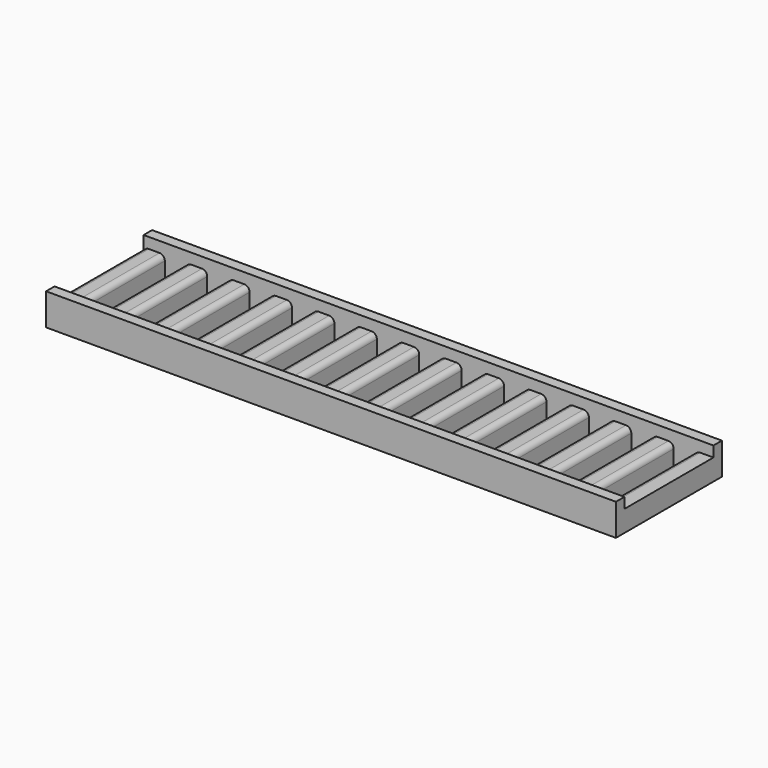
from build123d import *

# Parameters (mm, degrees)
F0_W     = 107.5
F0_H     = 25
F0_W_2   = 4
F0_H_2   = 21
F1_DEPTH = 4
F2_R     = 1
F3_W     = 107.5
F3_H     = 2
F4_DEPTH = 2
F5_R     = 1


# Not quite as in the source:
# - a feature names something its author has since deleted; it is built from what else it names


with BuildPart() as f1:
    # F0 (on Top) → F1 (new body)
    with BuildSketch(Plane.XY):
        with Locations((53.75, 12.5)):
            Rectangle(F0_W, F0_H)
        with Locations((6, 12.5)):
            Rectangle(F0_W_2, F0_H_2, mode=Mode.SUBTRACT)
        with Locations((14, 12.5)):
            Rectangle(F0_W_2, F0_H_2, mode=Mode.SUBTRACT)
        with Locations((22, 12.5)):
            Rectangle(F0_W_2, F0_H_2, mode=Mode.SUBTRACT)
        with Locations((30, 12.5)):
            Rectangle(F0_W_2, F0_H_2, mode=Mode.SUBTRACT)
        with Locations((38, 12.5)):
            Rectangle(F0_W_2, F0_H_2, mode=Mode.SUBTRACT)
        with Locations((46, 12.5)):
            Rectangle(F0_W_2, F0_H_2, mode=Mode.SUBTRACT)
        with Locations((54, 12.5)):
            Rectangle(F0_W_2, F0_H_2, mode=Mode.SUBTRACT)
        with Locations((62, 12.5)):
            Rectangle(F0_W_2, F0_H_2, mode=Mode.SUBTRACT)
        with Locations((70, 12.5)):
            Rectangle(F0_W_2, F0_H_2, mode=Mode.SUBTRACT)
        with Locations((78, 12.5)):
            Rectangle(F0_W_2, F0_H_2, mode=Mode.SUBTRACT)
        with Locations((86, 12.5)):
            Rectangle(F0_W_2, F0_H_2, mode=Mode.SUBTRACT)
        with Locations((94, 12.5)):
            Rectangle(F0_W_2, F0_H_2, mode=Mode.SUBTRACT)
        with Locations((102, 12.5)):
            Rectangle(F0_W_2, F0_H_2, mode=Mode.SUBTRACT)
    extrude(amount=F1_DEPTH)

    # F2
    f2_edges = [f1.edges().sort_by_distance(p)[0] for p in [
        (8, 12.5, 4),
        (12, 12.5, 4),
        (16, 12.5, 4),
        (20, 12.5, 4),
        (24, 12.5, 4),
        (28, 12.5, 4),
        (32, 12.5, 4),
        (36, 12.5, 4),
        (40, 12.5, 4),
        (44, 12.5, 4),
        (48, 12.5, 4),
        (52, 12.5, 4),
        (56, 12.5, 4),
        (60, 12.5, 4),
        (64, 12.5, 4),
        (68, 12.5, 4),
        (72, 12.5, 4),
        (76, 12.5, 4),
        (80, 12.5, 4),
        (84, 12.5, 4),
        (88, 12.5, 4),
        (92, 12.5, 4),
        (96, 12.5, 4),
        (100, 12.5, 4),
        (104, 12.5, 4),
    ]]
    fillet(f2_edges, radius=F2_R)

    # F3 (on face) → F4 (join)
    with BuildSketch(Plane.XY.offset(4)):
        with Locations((53.75, 1)):
            Rectangle(F3_W, F3_H)
        with Locations((53.75, 24)):
            Rectangle(F3_W, F3_H)
    extrude(amount=F4_DEPTH)

    # F5
    f5_edges = [f1.edges().sort_by_distance(p)[0] for p in [
        (4, 12.5, 4),
        (0, 12.5, 4),
    ]]
    fillet(f5_edges, radius=F5_R)


solid = f1.part
